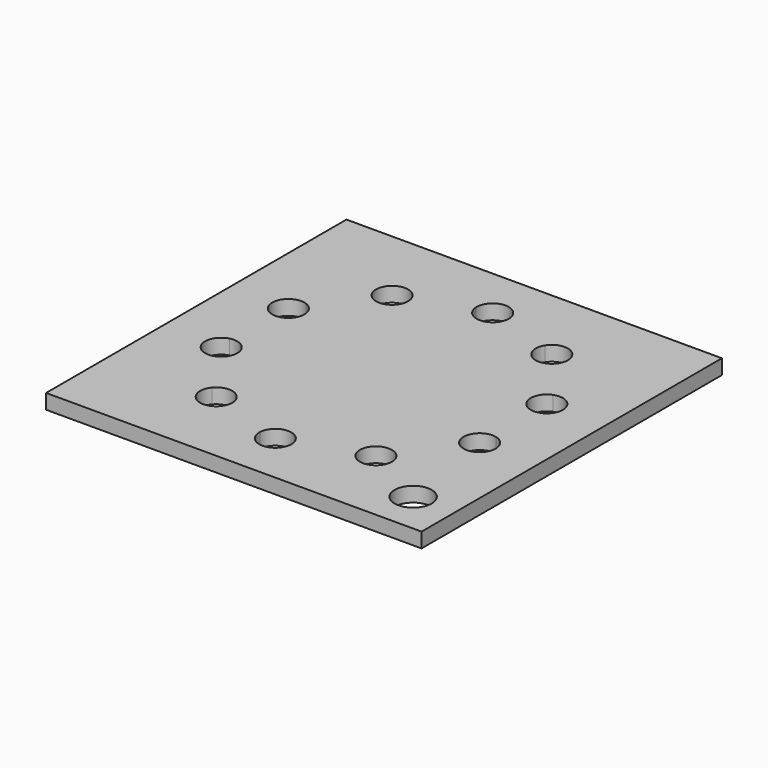
from build123d import *

# Parameters (mm, degrees)
F0_W     = 76
F0_H     = 76
F1_DEPTH = 3
F3_DEPTH = 25
F4_R     = 3.75
F5_DEPTH = 25


with BuildPart() as f1:
    # F0 (on Top) → F1 (new body)
    with BuildSketch(Plane.XY):
        Rectangle(F0_W, F0_H)
    extrude(amount=F1_DEPTH)

    # F2 (on face) → F3 (cut)
    with BuildSketch(Plane.XY.offset(3)):
        with BuildLine():
            ThreePointArc((24.9688578028, 11.5241546337), (23.0631205202, 7.4936621136), (26.9739584315, 5.3530894386))
            ThreePointArc((26.9739584315, 5.3530894386), (26.1540541981, 8.4979673453), (24.9688578028, 11.5241546337))
        make_face()
        with BuildLine():
            ThreePointArc((24.9688578028, 11.5241546337), (26.1540541981, 8.4979673453), (26.9739584315, 5.3530894386))
            ThreePointArc((26.9739584315, 5.3530894386), (28.7257451553, 6.5107819939), (29.4040541981, 8.4979673453))
            ThreePointArc((29.4040541981, 8.4979673453), (27.9858035963, 11.1825891329), (24.9688578028, 11.5241546337))
        make_face()
        with BuildLine():
            ThreePointArc((29.4040541981, -8.4979673453), (28.7257451553, -6.5107819939), (26.9739584315, -5.3530894386))
            ThreePointArc((26.9739584315, -5.3530894386), (26.1540541981, -8.4979673453), (24.9688578028, -11.5241546337))
            ThreePointArc((24.9688578028, -11.5241546337), (27.9858035963, -11.1825891329), (29.4040541981, -8.4979673453))
        make_face()
        with BuildLine():
            ThreePointArc((24.9688578028, -11.5241546337), (26.1540541981, -8.4979673453), (26.9739584315, -5.3530894386))
            ThreePointArc((26.9739584315, -5.3530894386), (23.0631205202, -7.4936621136), (24.9688578028, -11.5241546337))
        make_face()
        with BuildLine():
            ThreePointArc((13.4265021538, 23.9995633276), (14.2537923681, 19.6186621136), (18.6759237504, 20.1856352902))
            ThreePointArc((18.6759237504, 20.1856352902), (16.164094438, 22.2479673453), (13.4265021538, 23.9995633276))
        make_face()
        with BuildLine():
            ThreePointArc((13.4265021538, 23.9995633276), (16.164094438, 22.2479673453), (18.6759237504, 20.1856352902))
            ThreePointArc((18.6759237504, 20.1856352902), (19.2239919253, 21.1527379778), (19.414094438, 22.2479673453))
            ThreePointArc((19.414094438, 22.2479673453), (17.0765978836, 25.3672360836), (13.4265021538, 23.9995633276))
        make_face()
        with BuildLine():
            ThreePointArc((19.414094438, -22.2479673453), (19.2239919253, -21.1527379778), (18.6759237504, -20.1856352902))
            ThreePointArc((18.6759237504, -20.1856352902), (16.164094438, -22.2479673453), (13.4265021538, -23.9995633276))
            ThreePointArc((13.4265021538, -23.9995633276), (17.0765978836, -25.3672360836), (19.414094438, -22.2479673453))
        make_face()
        with BuildLine():
            ThreePointArc((13.4265021538, -23.9995633276), (16.164094438, -22.2479673453), (18.6759237504, -20.1856352902))
            ThreePointArc((18.6759237504, -20.1856352902), (14.2537923681, -19.6186621136), (13.4265021538, -23.9995633276))
        make_face()
        with BuildLine():
            ThreePointArc((-3.244320968, 27.3079545455), (0, 24.25), (3.244320968, 27.3079545455))
            ThreePointArc((3.244320968, 27.3079545455), (0, 27.5), (-3.244320968, 27.3079545455))
        make_face()
        with BuildLine():
            ThreePointArc((-3.244320968, 27.3079545455), (0, 27.5), (3.244320968, 27.3079545455))
            ThreePointArc((3.244320968, 27.3079545455), (3.2485799318, 27.4039352978), (3.25, 27.5))
            ThreePointArc((3.25, 27.5), (-0.0960647022, 30.7485799318), (-3.244320968, 27.3079545455))
        make_face()
        with BuildLine():
            ThreePointArc((3.25, -27.5), (3.2485799318, -27.4039352978), (3.244320968, -27.3079545455))
            ThreePointArc((3.244320968, -27.3079545455), (0, -27.5), (-3.244320968, -27.3079545455))
            ThreePointArc((-3.244320968, -27.3079545455), (-0.0960647022, -30.7485799318), (3.25, -27.5))
        make_face()
        with BuildLine():
            ThreePointArc((-3.244320968, -27.3079545455), (0, -27.5), (3.244320968, -27.3079545455))
            ThreePointArc((3.244320968, -27.3079545455), (0, -24.25), (-3.244320968, -27.3079545455))
        make_face()
        with BuildLine():
            ThreePointArc((-12.914094438, 22.2479673453), (-13.0448256997, 23.1604707908), (-13.4265021538, 23.9995633276))
            ThreePointArc((-13.4265021538, 23.9995633276), (-16.164094438, 22.2479673453), (-18.6759237504, 20.1856352902))
            ThreePointArc((-18.6759237504, 20.1856352902), (-15.0688650706, 19.188069858), (-12.914094438, 22.2479673453))
        make_face()
        with BuildLine():
            ThreePointArc((-18.6759237504, 20.1856352902), (-16.164094438, 22.2479673453), (-13.4265021538, 23.9995633276))
            ThreePointArc((-13.4265021538, 23.9995633276), (-18.074396508, 24.877272577), (-18.6759237504, 20.1856352902))
        make_face()
        with BuildLine():
            ThreePointArc((-18.6759237504, -20.1856352902), (-18.074396508, -24.877272577), (-13.4265021538, -23.9995633276))
            ThreePointArc((-13.4265021538, -23.9995633276), (-16.164094438, -22.2479673453), (-18.6759237504, -20.1856352902))
        make_face()
        with BuildLine():
            ThreePointArc((-18.6759237504, -20.1856352902), (-16.164094438, -22.2479673453), (-13.4265021538, -23.9995633276))
            ThreePointArc((-13.4265021538, -23.9995633276), (-13.0448256997, -23.1604707908), (-12.914094438, -22.2479673453))
            ThreePointArc((-12.914094438, -22.2479673453), (-15.0688650706, -19.188069858), (-18.6759237504, -20.1856352902))
        make_face()
        with BuildLine():
            ThreePointArc((-22.9040541981, 8.4979673453), (-23.4694324105, 10.3297167435), (-24.9688578028, 11.5241546337))
            ThreePointArc((-24.9688578028, 11.5241546337), (-26.1540541981, 8.4979673453), (-26.9739584315, 5.3530894386))
            ThreePointArc((-26.9739584315, 5.3530894386), (-24.1668688467, 5.9262763881), (-22.9040541981, 8.4979673453))
        make_face()
        with BuildLine():
            ThreePointArc((-26.9739584315, 5.3530894386), (-26.1540541981, 8.4979673453), (-24.9688578028, 11.5241546337))
            ThreePointArc((-24.9688578028, 11.5241546337), (-29.2449878761, 9.502272577), (-26.9739584315, 5.3530894386))
        make_face()
        with BuildLine():
            ThreePointArc((-26.9739584315, -5.3530894386), (-29.2449878761, -9.502272577), (-24.9688578028, -11.5241546337))
            ThreePointArc((-24.9688578028, -11.5241546337), (-26.1540541981, -8.4979673453), (-26.9739584315, -5.3530894386))
        make_face()
        with BuildLine():
            ThreePointArc((-26.9739584315, -5.3530894386), (-26.1540541981, -8.4979673453), (-24.9688578028, -11.5241546337))
            ThreePointArc((-24.9688578028, -11.5241546337), (-23.4694324105, -10.3297167435), (-22.9040541981, -8.4979673453))
            ThreePointArc((-22.9040541981, -8.4979673453), (-24.1668688467, -5.9262763881), (-26.9739584315, -5.3530894386))
        make_face()
    extrude(amount=-F3_DEPTH, mode=Mode.SUBTRACT)

    # F4 (on face) → F5 (cut)
    with BuildSketch(Plane.XY.offset(3)):
        with Locations((29.5, -29.5)):
            Circle(F4_R)
    extrude(amount=-F5_DEPTH, mode=Mode.SUBTRACT)


solid = f1.part
